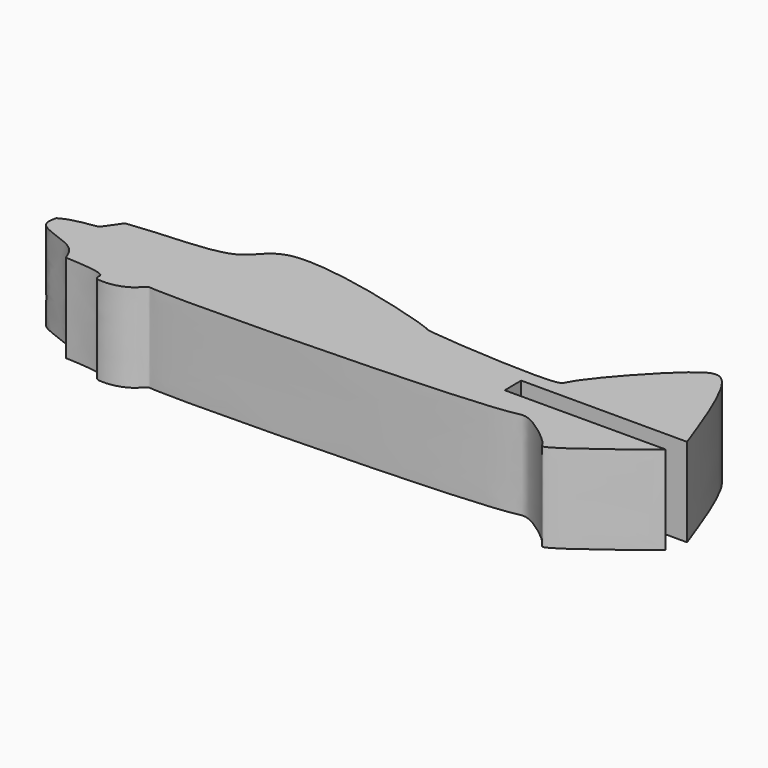
from build123d import *

# Parameters (mm, degrees)
F1_DEPTH = 18.7


with BuildPart() as f1:
    # F0 (on Top) → F1 (new body)
    with BuildSketch(Plane.XY):
        with BuildLine():
            add(Edge.make_bspline(
                [(-59.0569749475, 5.6584109552), (-49.5342656666, 6.8617920581), (-35.8377748643, 5.9807723499), (-32.8955110008, 18.374842932), (4.1516991759, 7.6361436104), (3.1341130081, 6.7788110675), (33.4644857612, 4.593264758), (32.9304993939, 7.6650975099), (47.0177142926, 23.7469349464), (54.1062876892, 25.9705380057), (60.3101640298, 7.5653437461), (62.1775598622, 2.6169322648)],
                knots=[0, 0, 0, 0, 0.0704652856, 0.1151765677, 0.2022320057, 0.2196207652, 0.2984568882, 0.3232517394, 0.3912680681, 0.4270669045, 0.4894185359, 0.4894185359, 0.4894185359, 0.4894185359], degree=3))
            add(Edge.make_bspline(
                [(-59.0569749475, 5.6584109552), (-61.6470714196, 2.2157883375), (-60.6743437248, 1.9244718037), (-66.8684896329, 1.3664782498), (-69.0759941936, 0)],
                knots=[0, 0, 0, 0, 0.4547450823, 1, 1, 1, 1], degree=3))
            add(Edge.make_bspline(
                [(-69.0759941936, 0), (-69.3788101739, -1.1783828473), (-69.8261399485, -3.9587908232), (-60.6959776767, -5.7092868497), (-59.5250335128, -8.7119018904), (-59.0307191014, -10.0178774446)],
                knots=[0, 0, 0, 0, 0.2642250224, 0.6877674352, 1, 1, 1, 1], degree=3))
            add(Edge.make_bspline(
                [(61.0633843308, -1.7152679098), (56.7431976085, -5.3030378612), (44.3625908851, -14.8355506131), (44.3456154781, -12.4734236778), (36.3078073079, -6.1540606425), (32.5025622398, -7.8491580238), (0.9720994688, -9.5558607176), (-40.314506836, -10.1098663132), (-41.996994883, -9.4756719581), (-44.3149303482, -12.8199559019), (-51.5631544474, -13.2743806674), (-49.3621790744, -10.1875372552), (-58.816473348, -10.0654157712), (-59.0307191014, -10.0178774446)],
                knots=[0.5262904111, 0.5262904111, 0.5262904111, 0.5262904111, 0.5845122047, 0.6007471474, 0.6464191733, 0.6752026649, 0.7615315554, 0.8575421685, 0.8732136115, 0.9023140778, 0.9379261728, 0.9554425291, 0.9986146344, 0.9986146344, 0.9986146344, 0.9986146344], degree=3))
            Line((61.0633843308, -1.7152679098), (27.176482603, -1.7873676261))
            Line((27.176482603, -1.7873676261), (27.1043330431, 2.6169322648))
            Line((27.1043330431, 2.6169322648), (42.1066259529, 2.6169322648))
            Line((42.1066259529, 2.6169322648), (62.1775598622, 2.6169322648))
        make_face()
    extrude(amount=F1_DEPTH)


solid = f1.part
